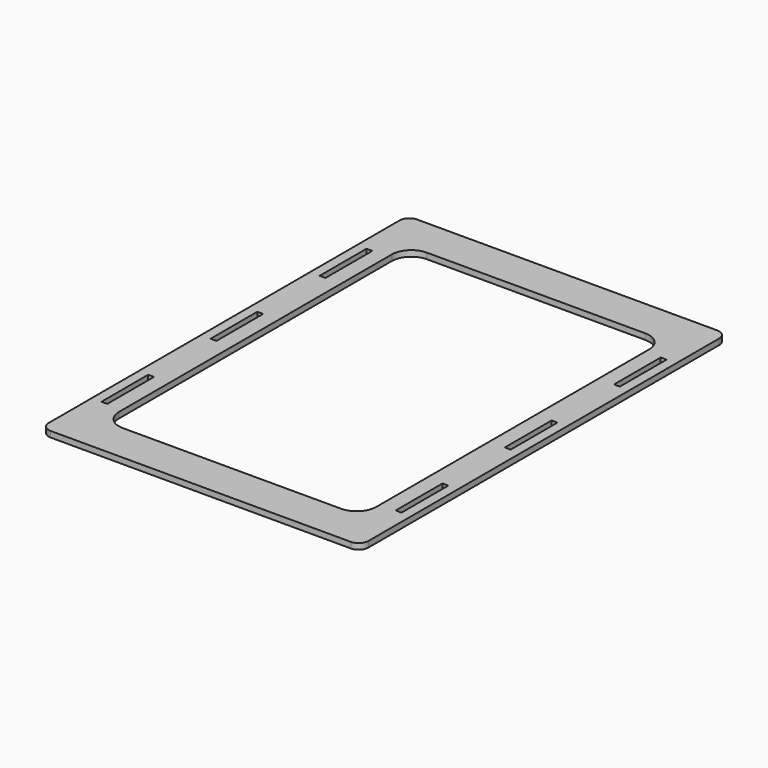
from build123d import *

# Parameters (mm, degrees)
F0_W     = 164
F0_H     = 235
F0_W_2   = 3
F0_H_2   = 30
F0_W_3   = 132
F0_H_3   = 195
F1_DEPTH = 3
F2_R     = 5
F3_R     = 10


with BuildPart() as f1:
    # F0 (on Top) → F1 (new body)
    with BuildSketch(Plane.XY):
        with Locations((77, 112.5)):
            Rectangle(F0_W, F0_H)
        with Locations((1.5, 42.5)):
            Rectangle(F0_W_2, F0_H_2, mode=Mode.SUBTRACT)
        with Locations((152.5, 42.5)):
            Rectangle(F0_W_2, F0_H_2, mode=Mode.SUBTRACT)
        with Locations((1.5, 112.5)):
            Rectangle(F0_W_2, F0_H_2, mode=Mode.SUBTRACT)
        with Locations((1.5, 182.5)):
            Rectangle(F0_W_2, F0_H_2, mode=Mode.SUBTRACT)
        with Locations((77, 112.5)):
            Rectangle(F0_W_3, F0_H_3, mode=Mode.SUBTRACT)
        with Locations((152.5, 112.5)):
            Rectangle(F0_W_2, F0_H_2, mode=Mode.SUBTRACT)
        with Locations((152.5, 182.5)):
            Rectangle(F0_W_2, F0_H_2, mode=Mode.SUBTRACT)
    extrude(amount=F1_DEPTH)

    # F2
    f2_edges = [f1.edges().sort_by_distance(p)[0] for p in [
        (-5, 230, 1.5),
        (159, 230, 1.5),
        (159, -5, 1.5),
        (-5, -5, 1.5),
    ]]
    fillet(f2_edges, radius=F2_R)

    # F3
    f3_edges = [f1.edges().sort_by_distance(p)[0] for p in [
        (11, 210, 1.5),
        (143, 210, 1.5),
        (143, 15, 1.5),
        (11, 15, 1.5),
    ]]
    fillet(f3_edges, radius=F3_R)


solid = f1.part
